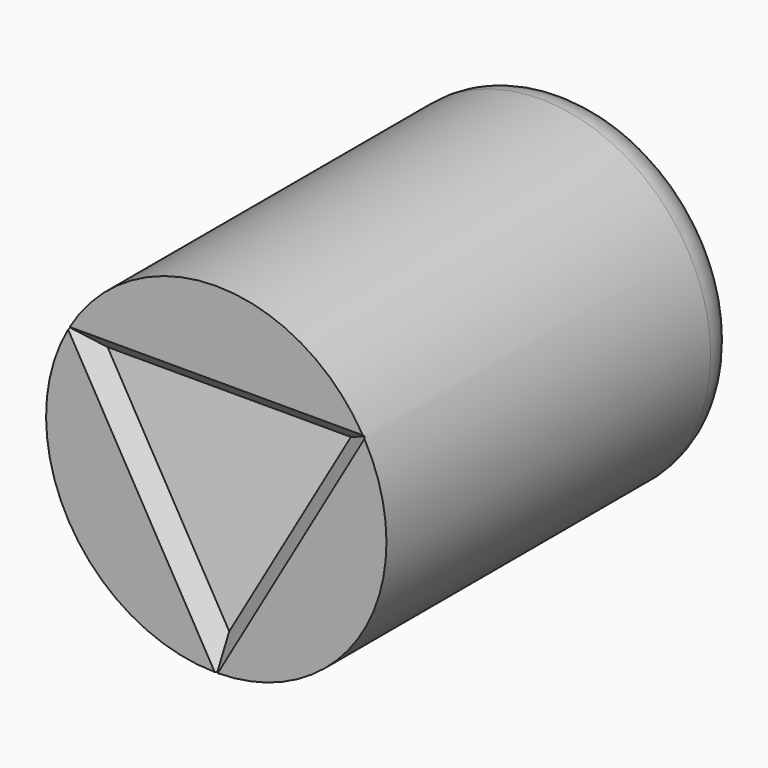
from build123d import *

# Parameters (mm, degrees)
F0_R         = 10.5
F1_DEPTH     = 25
F2_R         = 10.5
F3_DEPTH     = 2.5
F4_R         = 2.49999
F5_T4_DEPTH  = 20.1544729749
F5_T10_DEPTH = 20.1544729749
F5_T16_DEPTH = 20.1544729749
F5_T23_DEPTH = 20.1544729749
F5_T27_DEPTH = 20.1544729749
F5_T34_DEPTH = 20.1544729749
F5_T38_DEPTH = 20.1544729749
F5_T45_DEPTH = 20.1544729749
F5_T49_DEPTH = 20.1544729749


# Not quite as in the source:
# - a fillet or chamfer that OpenCascade refuses, or shapes differently, is made with other operations: its cross-section is extruded or revolved along the edge and cut away or added
# - a fillet or chamfer is up to 0.001 mm smaller than in the source, because OpenCascade refuses the exact size


with BuildPart() as f1:
    # F0 (on Front) → F1 (new body)
    with BuildSketch(Plane.XZ):
        Circle(F0_R)
        Polygon((0, -8.6666666667), (-7.5055534995, 4.3333333333), (7.5055534995, 4.3333333333), align=None, mode=Mode.SUBTRACT)
    extrude(amount=F1_DEPTH)

    # F2 (on Front) → F3 (join)
    with BuildSketch(Plane.XZ):
        Circle(F2_R)
    extrude(amount=-F3_DEPTH)

    # F4 (radius 2.5 in the source; OpenCascade refuses exactly that, so slightly less here)
    f4_edges = [f1.edges().sort_by_distance(p)[0] for p in [
        (-10.5, 2.5, 0),
    ]]
    fillet(f4_edges, radius=F4_R)

    # F5: chamfer of 1 on 3 edges, made by hand


with BuildPart() as f5_tool2:
    # F5_s3 → F5_t4 (new body)
    with BuildSketch(Plane(origin=(5.0386182437, 0, -8.7271427981), x_dir=(0, 1, 0), z_dir=(-0.5, 0, 0.8660254038))):
        Polygon((-25, 5.3333333333), (-24, 4.3333333333), (-25, 4.3333333333), align=None)
    extrude(amount=F5_T4_DEPTH)

    split(bisect_by=Plane(origin=(3.7527767497, 0, -2.1666666667), x_dir=(0, 1, 0), z_dir=(-0.8660254038, 0, 0.5)), keep=Keep.TOP)

    split(bisect_by=Plane.XY.offset(4.3333333333), keep=Keep.BOTTOM)


with BuildPart() as f1_1:
    add(f1.part)

    # F5_t1: cut F5_tool2
    add(f5_tool2.part, mode=Mode.SUBTRACT)


with BuildPart() as f5_tool8:
    # F5_s9 → F5_t10 (new body)
    with BuildSketch(Plane.YZ.offset(-10.0772364874)):
        Polygon((-25, 5.3333333333), (-24, 4.3333333333), (-25, 4.3333333333), align=None)
    extrude(amount=F5_T10_DEPTH)

    split(bisect_by=Plane(origin=(3.7527767497, 0, -2.1666666667), x_dir=(0, 1, 0), z_dir=(-0.8660254038, 0, 0.5)), keep=Keep.TOP)

    split(bisect_by=Plane(origin=(-3.7527767497, 0, -2.1666666667), x_dir=(0, 1, 0), z_dir=(0.8660254038, 0, 0.5)), keep=Keep.TOP)


with BuildPart() as f1_2:
    add(f1_1.part)

    # F5_t7: cut F5_tool8
    add(f5_tool8.part, mode=Mode.SUBTRACT)


with BuildPart() as f5_tool14:
    # F5_s15 → F5_t16 (new body)
    with BuildSketch(Plane(origin=(5.0386182437, 0, 8.7271427981), x_dir=(0, 1, 0), z_dir=(-0.5, 0, -0.8660254038))):
        Polygon((-25, 5.3333333333), (-24, 4.3333333333), (-25, 4.3333333333), align=None)
    extrude(amount=F5_T16_DEPTH)

    split(bisect_by=Plane.XY.offset(4.3333333333), keep=Keep.BOTTOM)

    split(bisect_by=Plane(origin=(-3.7527767497, 0, -2.1666666667), x_dir=(0, 1, 0), z_dir=(0.8660254038, 0, 0.5)), keep=Keep.TOP)


with BuildPart() as f1_3:
    add(f1_2.part)

    # F5_t13: cut F5_tool14
    add(f5_tool14.part, mode=Mode.SUBTRACT)


with BuildPart() as f5_tool21:
    # F5_s22 → F5_t23 (new body)
    with BuildSketch(Plane(origin=(5.0386182437, 0, 8.7271427981), x_dir=(0, 1, 0), z_dir=(-0.5, 0, -0.8660254038))):
        Polygon((-25, 5.3333333333), (-24, 4.3333333333), (-25, 4.3333333333), align=None)
    extrude(amount=F5_T23_DEPTH)

    split(bisect_by=Plane(origin=(-3.7527767497, 0, -2.1666666667), x_dir=(0, 1, 0), z_dir=(-0.8660254038, 0, -0.5)), keep=Keep.TOP)


with BuildPart() as f5_tool25:
    # F5_s26 → F5_t27 (new body)
    with BuildSketch(Plane(origin=(5.0386182437, 0, -8.7271427981), x_dir=(0, 1, 0), z_dir=(-0.5, 0, 0.8660254038))):
        Polygon((-25, 5.3333333333), (-24, 4.3333333333), (-25, 4.3333333333), align=None)
    extrude(amount=F5_T27_DEPTH)

    split(bisect_by=Plane(origin=(3.7527767497, 0, -2.1666666667), x_dir=(0, 1, 0), z_dir=(0.8660254038, 0, -0.5)), keep=Keep.TOP)


with BuildPart() as f5_tool21_1:
    add(f5_tool21.part)

    # F5_t29: intersect F5_tool25
    add(f5_tool25.part, mode=Mode.INTERSECT)


with BuildPart() as f1_4:
    add(f1_3.part)

    # F5_t19: cut F5_tool21
    add(f5_tool21_1.part, mode=Mode.SUBTRACT)


with BuildPart() as f5_tool32:
    # F5_s33 → F5_t34 (new body)
    with BuildSketch(Plane(origin=(5.0386182437, 0, -8.7271427981), x_dir=(0, 1, 0), z_dir=(-0.5, 0, 0.8660254038))):
        Polygon((-25, 5.3333333333), (-24, 4.3333333333), (-25, 4.3333333333), align=None)
    extrude(amount=F5_T34_DEPTH)

    split(bisect_by=Plane.XY.offset(4.3333333333), keep=Keep.TOP)


with BuildPart() as f5_tool36:
    # F5_s37 → F5_t38 (new body)
    with BuildSketch(Plane.YZ.offset(-10.0772364874)):
        Polygon((-25, 5.3333333333), (-24, 4.3333333333), (-25, 4.3333333333), align=None)
    extrude(amount=F5_T38_DEPTH)

    split(bisect_by=Plane(origin=(-3.7527767497, 0, -2.1666666667), x_dir=(0, 1, 0), z_dir=(-0.8660254038, 0, -0.5)), keep=Keep.TOP)


with BuildPart() as f5_tool32_1:
    add(f5_tool32.part)

    # F5_t40: intersect F5_tool36
    add(f5_tool36.part, mode=Mode.INTERSECT)


with BuildPart() as f1_5:
    add(f1_4.part)

    # F5_t30: cut F5_tool32
    add(f5_tool32_1.part, mode=Mode.SUBTRACT)


with BuildPart() as f5_tool43:
    # F5_s44 → F5_t45 (new body)
    with BuildSketch(Plane(origin=(5.0386182437, 0, 8.7271427981), x_dir=(0, 1, 0), z_dir=(-0.5, 0, -0.8660254038))):
        Polygon((-25, 5.3333333333), (-24, 4.3333333333), (-25, 4.3333333333), align=None)
    extrude(amount=F5_T45_DEPTH)

    split(bisect_by=Plane.XY.offset(4.3333333333), keep=Keep.TOP)


with BuildPart() as f5_tool47:
    # F5_s48 → F5_t49 (new body)
    with BuildSketch(Plane.YZ.offset(-10.0772364874)):
        Polygon((-25, 5.3333333333), (-24, 4.3333333333), (-25, 4.3333333333), align=None)
    extrude(amount=F5_T49_DEPTH)

    split(bisect_by=Plane(origin=(3.7527767497, 0, -2.1666666667), x_dir=(0, 1, 0), z_dir=(0.8660254038, 0, -0.5)), keep=Keep.TOP)


with BuildPart() as f5_tool43_1:
    add(f5_tool43.part)

    # F5_t51: intersect F5_tool47
    add(f5_tool47.part, mode=Mode.INTERSECT)


with BuildPart() as f1_6:
    add(f1_5.part)

    # F5_t41: cut F5_tool43
    add(f5_tool43_1.part, mode=Mode.SUBTRACT)


solid = f1_6.part
